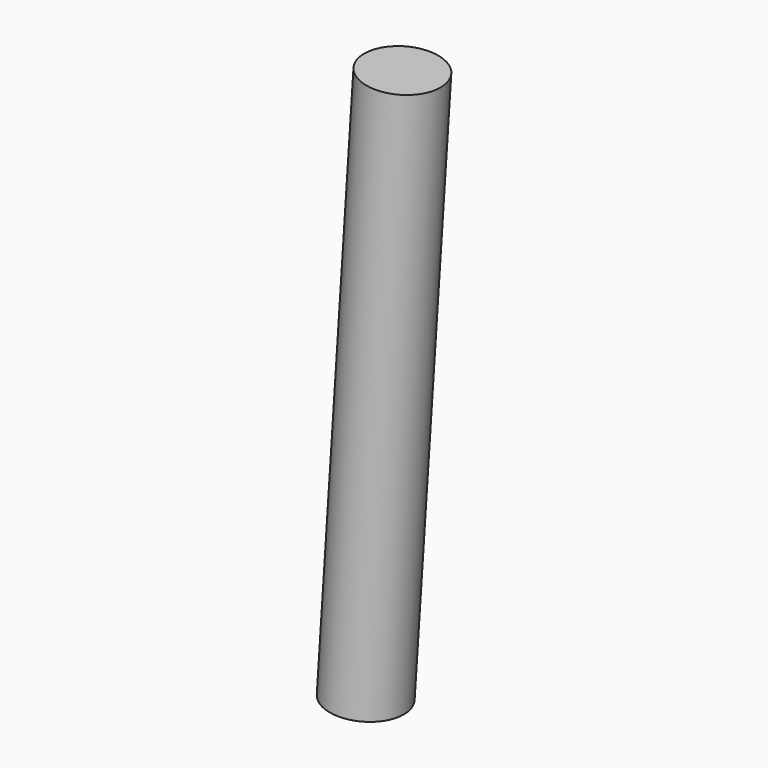
from build123d import *

# Parameters (mm, degrees)
F2_R = 50.8


with BuildPart() as f3:
    # F3: sweep along a path in F0
    with BuildLine(Plane.XZ) as f3_path:
        Line((201.2927353119, -134.5406058412), (152.6, -882.7))
    # F2 (on face) → F3 (sweep)
    with BuildSketch(Plane(origin=(-32.2167412585, 0, -495.007262733), x_dir=(0.9978887822, 0, -0.0649459657), z_dir=(-0.0649459657, 0, -0.9978887822))):
        with Locations((209.6056320663, 0)):
            Circle(F2_R)
    sweep(path=f3_path.line)


solid = f3.part
